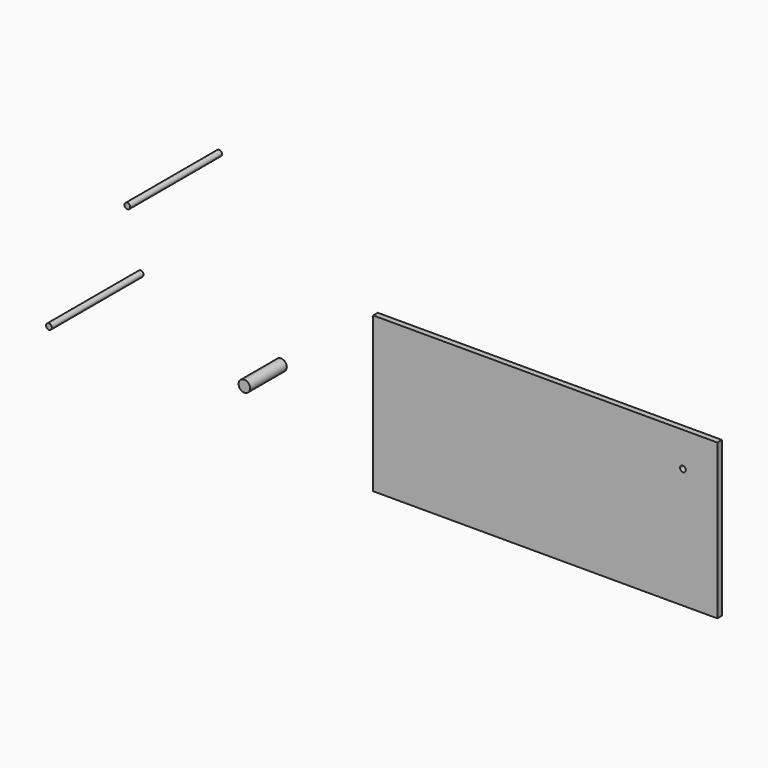
from build123d import *

# Parameters (mm, degrees)
F0_W     = 762
F0_H     = 342.7822869062
F0_R     = 6.35
F1_DEPTH = 12.7
F2_R     = 12.7
F3_DEPTH = 101.6
F4_DEPTH = 254


# Not quite as in the source:
# - the program builds the solid bodies; features that only make, move or delete a surface that nothing else refers to are left out


with BuildPart() as f1:
    # F0 (on Front) → F1 (new body)
    with BuildSketch(Plane.XZ):
        with Locations((-256.4684061597, 0)):
            Rectangle(F0_W, F0_H)
        with Locations((48.3315938403, 95.1911434531)):
            Circle(F0_R, mode=Mode.SUBTRACT)
    extrude(amount=F1_DEPTH)


with BuildPart() as f3:
    # F2 (on Front) → F3 (new body)
    with BuildSketch(Plane.XZ):
        with Locations((-851.6189455986, 0)):
            Circle(F2_R)
    extrude(amount=F3_DEPTH)


with BuildPart() as f4:
    # F0 (on Front) → F4 (new body)
    with BuildSketch(Plane.XZ):
        with Locations((-988.6716604233, 368.4581816196)):
            Circle(F0_R)
    extrude(amount=F4_DEPTH)


with BuildPart() as f4b:
    # F0 (on Front) → F4, piece 2 (new body)
    with BuildSketch(Plane.XZ):
        with Locations((-1162.283539772, 76.9616737962)):
            Circle(F0_R)
    extrude(amount=F4_DEPTH)


solid = Compound([f1.part, f3.part, f4.part, f4b.part])
